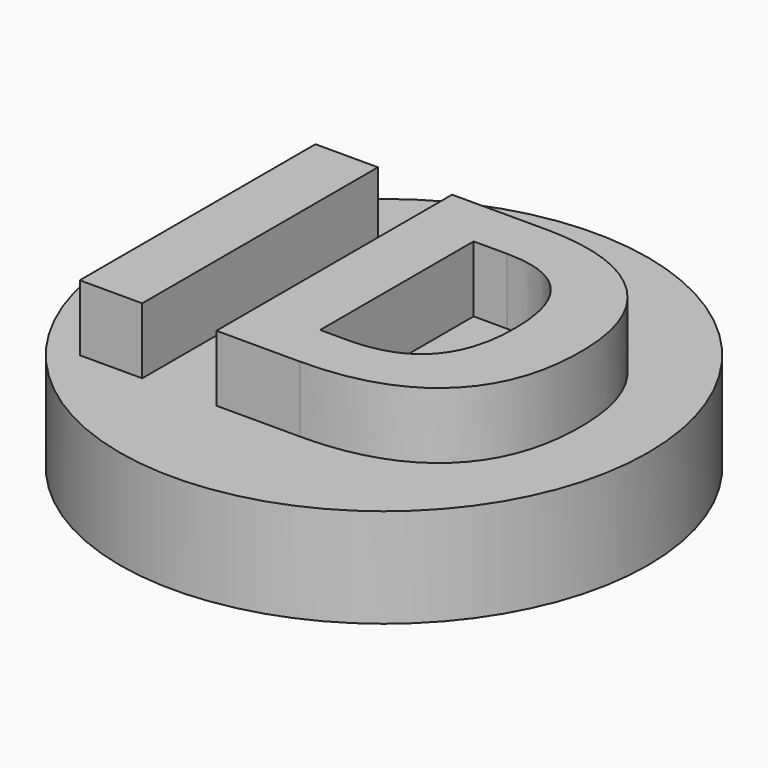
from build123d import *

# Parameters (mm, degrees)
F0_R         = 8
F0_W         = 1.892578125
F0_H         = 8.923828125
F1_DEPTH     = 3
F0_TEXT_SIZE = 12.5
F2_DEPTH     = 5


# Not quite as in the source:
# - Text() gives the source's letters only with a copy of the font that has no kerning and outlines rounded to 1/6400 em; it was checked with that copy


with BuildPart() as f1:
    # F0 (on Top) → F1 (new body)
    with BuildSketch(Plane.XY):
        Circle(F0_R)
        with Locations((-4.6689453125, -0.0380859375)):
            Rectangle(F0_W, F0_H, mode=Mode.SUBTRACT)
        with BuildLine():
            add(Edge.make_bspline(
                [(4.71875, 3.2705078125), (5.927734375, 2.1171875), (5.927734375, 0.046875)],
                knots=[0, 0, 0, 1, 1, 1], degree=2))
            add(Edge.make_bspline(
                [(5.927734375, 0.046875), (5.927734375, -2.15625), (4.6728515625, -3.328125)],
                knots=[0, 0, 0, 1, 1, 1], degree=2))
            add(Edge.make_bspline(
                [(4.6728515625, -3.328125), (3.41796875, -4.5), (1.05078125, -4.5)],
                knots=[0, 0, 0, 1, 1, 1], degree=2))
            Line((1.05078125, -4.5), (-1.4765625, -4.5))
            Line((-1.4765625, -4.5), (-1.4765625, 4.423828125))
            Line((-1.4765625, 4.423828125), (1.32421875, 4.423828125))
            add(Edge.make_bspline(
                [(1.32421875, 4.423828125), (3.509765625, 4.423828125), (4.71875, 3.2705078125)],
                knots=[0, 0, 0, 1, 1, 1], degree=2))
        make_face(mode=Mode.SUBTRACT)
    extrude(amount=F1_DEPTH)



with BuildPart() as f1b:
    # F0 (on Top) → F1, piece 2 (new body)
    with BuildSketch(Plane.XY):
        with BuildLine():
            add(Edge.make_bspline(
                [(1.2265625, -2.9375), (3.9609375, -2.9375), (3.9609375, -0.001953125)],
                knots=[0, 0, 0, 1, 1, 1], degree=2))
            add(Edge.make_bspline(
                [(3.9609375, -0.001953125), (3.9609375, 2.873046875), (1.421875, 2.873046875)],
                knots=[0, 0, 0, 1, 1, 1], degree=2))
            Line((1.421875, 2.873046875), (0.416015625, 2.873046875))
            Line((0.416015625, 2.873046875), (0.416015625, -2.9375))
            Line((0.416015625, -2.9375), (1.2265625, -2.9375))
        make_face()
    extrude(amount=F1_DEPTH)


with BuildPart() as f1_1:
    add(f1.part)

    add(f1b.part)  # F2 merges F1b
    # F0 (on Top) → F2 (join)
    with BuildSketch(Plane.XY):
        with Locations((-6.73828125, -4.5)):
            Text('ID', F0_TEXT_SIZE, font='Open Sans', font_style=FontStyle.BOLD, text_align=(TextAlign.LEFT, TextAlign.BOTTOM))
    extrude(amount=F2_DEPTH)


solid = f1_1.part
